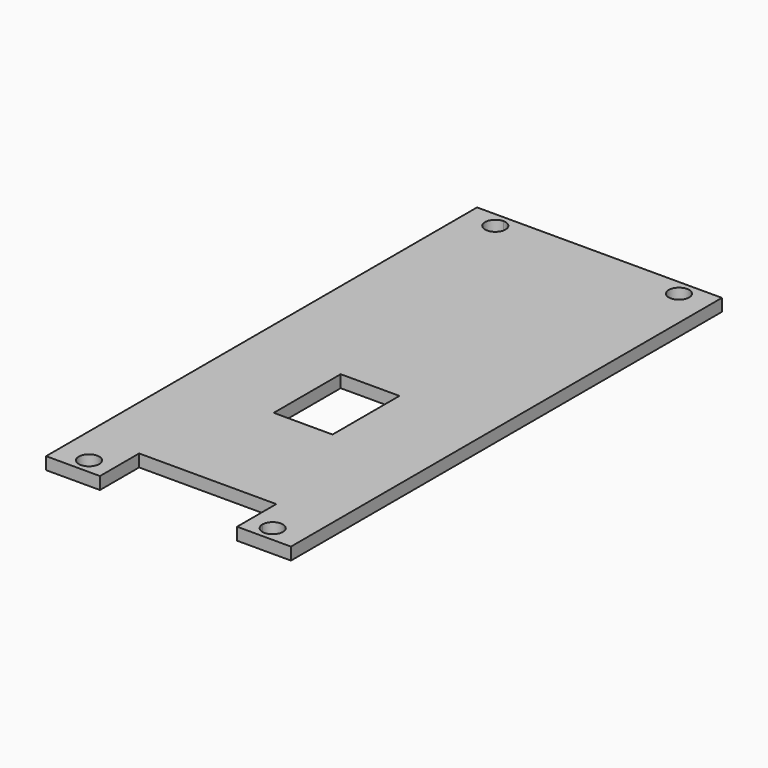
from build123d import *

# Parameters (mm, degrees)
F0_W             = 31.75
F0_H             = 63.5
F0_W_2           = 7.62
F0_H_2           = 10.8501603827
F1_DEPTH         = 1.6
F2_W             = 6.985
F2_H             = 1.6
F3_DEPTH         = 6.35
F5_DEPTH         = 25.4
F5_COPIES2_COUNT = 2
F5_COPIES2_PITCH = 70.023265


# Not quite as in the source:
# - a feature of the source that left no trace in its solid (it failed there, or was rolled back) is left out
# - a pattern or mirror of a feature is missing from the dataset's text; its kind, count and spacing are read off the source's solid
# - a feature names something its author has since deleted; it is built from what else it names


with BuildPart() as f1:
    # F0 (on Top) → F1 (new body)
    with BuildSketch(Plane.XY):
        with Locations((15.875, 31.75)):
            Rectangle(F0_W, F0_H)
        with Locations((15.875, 20.8916743286)):
            Rectangle(F0_W_2, F0_H_2, mode=Mode.SUBTRACT)
    extrude(amount=F1_DEPTH)

    # F2 (on face) → F3 (join)
    with BuildSketch(Plane.XZ):
        with Locations((3.4925, 0.8)):
            Rectangle(F2_W, F2_H)
        with Locations((28.2575, 0.8)):
            Rectangle(F2_W, F2_H)
    extrude(amount=F3_DEPTH)

    # F4 (on face) → F5 (cut)
    with BuildSketch(Plane.XY.offset(1.6)):
        with BuildLine():
            ThreePointArc((5.29375, -4.35), (3.0318335149, -3.4130835149), (3.96875, -5.675))
            Line((3.96875, -5.675), (3.96875, -4.35))
            Line((3.96875, -4.35), (5.29375, -4.35))
        make_face()
        with BuildLine():
            Line((3.96875, -4.35), (3.96875, -5.675))
            ThreePointArc((3.96875, -5.675), (4.9056664851, -5.2869164851), (5.29375, -4.35))
            Line((5.29375, -4.35), (3.96875, -4.35))
        make_face()
    f5 = extrude(amount=-F5_DEPTH, mode=Mode.SUBTRACT)

    # F5_copies: F5 across plane
    add(f5.mirror(Plane.ZX.offset(28.575)), mode=Mode.SUBTRACT)

    # F5_copies1: F5 across plane
    add(f5.mirror(Plane(origin=(15.875, 0, 0), x_dir=(0, 0, 1), z_dir=(1, 0, 0))), mode=Mode.SUBTRACT)

    # F5_copies2: F5 ×2
    with Locations(*[Vector(0.3400655477, 0.940401735, 0) * (i * F5_COPIES2_PITCH) for i in range(1, F5_COPIES2_COUNT)]):
        add(f5, mode=Mode.SUBTRACT)


solid = f1.part
